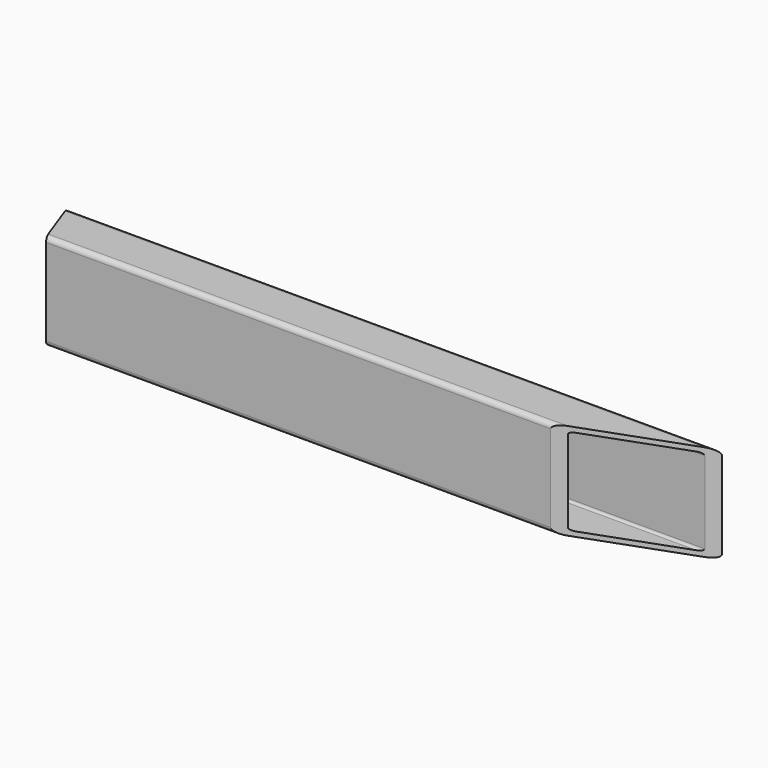
from build123d import *

# Parameters (mm, degrees)
F0_W     = 344.4875
F0_H     = 50.8
F1_DEPTH = 12.7
F2_T     = -2.54
F4_DEPTH = 50.801
F6_DEPTH = 50.801
F7_R     = 2.54
F8_R     = 1.27


# Not quite as in the source:
# - a feature names something its author has since deleted; it is built from what else it names


with BuildPart() as f1:
    # F0 (on Front) → F1 (new body, symmetric)
    with BuildSketch(Plane.XZ):
        Rectangle(F0_W, F0_H)
    extrude(amount=F1_DEPTH, both=True)

    # F2
    f2_openings = [f1.faces().sort_by_distance(p)[0] for p in [
        (-172.24375, 0, 0),
        (172.24375, 0, 0),
    ]]
    offset(amount=F2_T, openings=f2_openings)

    # F3 (on face) → F4 (cut, through all)
    with BuildSketch(Plane.XY.offset(25.4)):
        Polygon((-162.9989060496, -12.7), (-172.24375, 12.7), (-172.24375, -12.7), align=None)
    extrude(amount=-F4_DEPTH, mode=Mode.SUBTRACT)

    # F5 (on face) → F6 (cut, through all)
    with BuildSketch(Plane.XY.offset(25.4)):
        Polygon((172.24375, -12.7), (172.24375, 12.7), (102.4578235459, -12.7), align=None)
    extrude(amount=-F6_DEPTH, mode=Mode.SUBTRACT)

    # F7
    f7_edges = [f1.edges().sort_by_distance(p)[0] for p in [
        (-30.270541, -12.7, 25.4),
        (0, 12.7, 25.4),
        (0, 12.7, -25.4),
        (-30.270541, -12.7, -25.4),
    ]]
    fillet(f7_edges, radius=F7_R)

    # F8
    f8_edges = [f1.edges().sort_by_distance(p)[0] for p in [
        (-27.243487, -10.16, -22.86),
        (-27.243487, -10.16, 22.86),
        (-3.027054, 10.16, 22.86),
        (-3.027054, 10.16, -22.86),
    ]]
    fillet(f8_edges, radius=F8_R)


solid = f1.part
